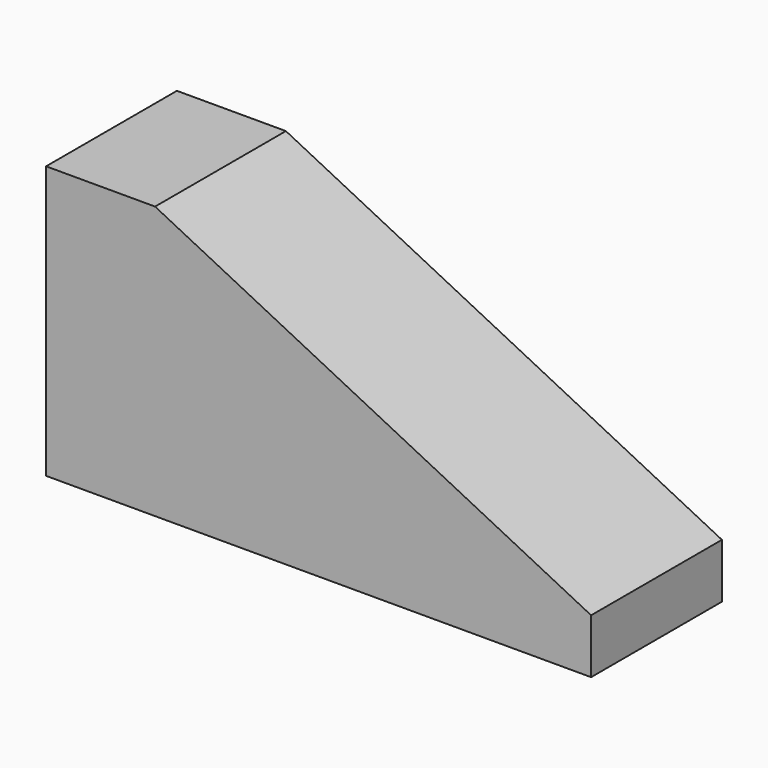
from build123d import *

# Parameters (mm, degrees)
F0_W     = 25.4
F0_H     = 63.5
F1_DEPTH = 38.1


# Not quite as in the source:
# - a feature names something its author has since deleted; it is built from what else it names


with BuildPart() as f1:
    # F0 (on Front) → F1 (new body)
    with BuildSketch(Plane.XZ):
        Polygon((-101.6, 63.5), (-101.6, 0), (-29.9632605165, 0), (0, 0), (0, 12.7), align=None)
        with Locations((-114.3, 31.75)):
            Rectangle(F0_W, F0_H)
    extrude(amount=F1_DEPTH)


solid = f1.part
